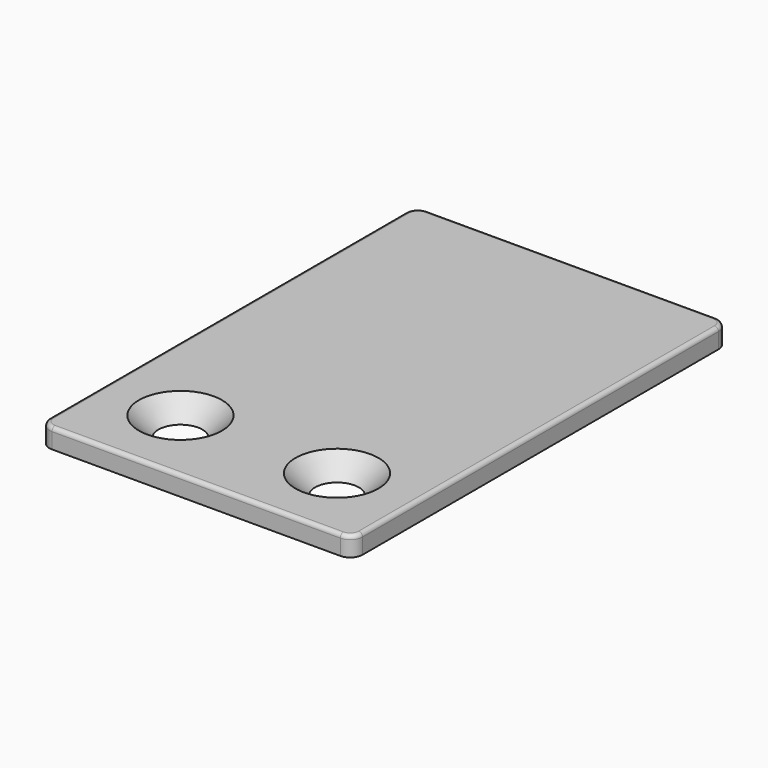
from build123d import *

# Parameters (mm, degrees)
F0_R     = 5
F1_DEPTH = 5
F2_R     = 1


# Not quite as in the source:
# - a fillet or chamfer that OpenCascade refuses, or shapes differently, is made with other operations: its cross-section is extruded or revolved along the edge and cut away or added


with BuildPart() as f1:
    # F0 (on Top) → F1 (new body)
    with BuildSketch(Plane.XY):
        with BuildLine():
            ThreePointArc((-40, -56.83), (-39.0715284964, -59.0715284964), (-36.83, -60))
            Line((-36.83, -60), (36.83, -60))
            ThreePointArc((36.83, -60), (39.0715284964, -59.0715284964), (40, -56.83))
            Line((40, -56.83), (40, 56.83))
            ThreePointArc((40, 56.83), (39.0715284964, 59.0715284964), (36.83, 60))
            Line((36.83, 60), (-36.83, 60))
            ThreePointArc((-36.83, 60), (-39.0715284964, 59.0715284964), (-40, 56.83))
            Line((-40, 56.83), (-40, -56.83))
        make_face()
        with Locations((-19.9999991059, -40.0115316966)):
            Circle(F0_R, mode=Mode.SUBTRACT)
        with Locations((20.0000008941, -40.0115316966)):
            Circle(F0_R, mode=Mode.SUBTRACT)
    extrude(amount=F1_DEPTH)

    # F2
    f2_edges = [f1.edges().sort_by_distance(p)[0] for p in [
        (-40, 0, 5),
    ]]
    fillet(f2_edges, radius=F2_R)

    # F3: chamfer of 5.6 on 2 edges, made by hand

    # F3_s1 → F3_t2 (revolve, cut)
    with BuildSketch(Plane.XZ.offset(40.0115316966)):
        Polygon((-9.3999991059, 5), (-14.9999991059, -0.6), (-14.9999991059, 5), align=None)
    revolve(axis=Axis((-19.9999991059, -40.0115316966, 5), (0, 0, 1)), mode=Mode.SUBTRACT)

    # F3_s3 → F3_t4 (revolve, cut)
    with BuildSketch(Plane.XZ.offset(40.0115316966)):
        Polygon((30.6000008941, 5), (25.0000008941, -0.6), (25.0000008941, 5), align=None)
    revolve(axis=Axis((20.0000008941, -40.0115316966, 5), (0, 0, 1)), mode=Mode.SUBTRACT)


solid = f1.part
